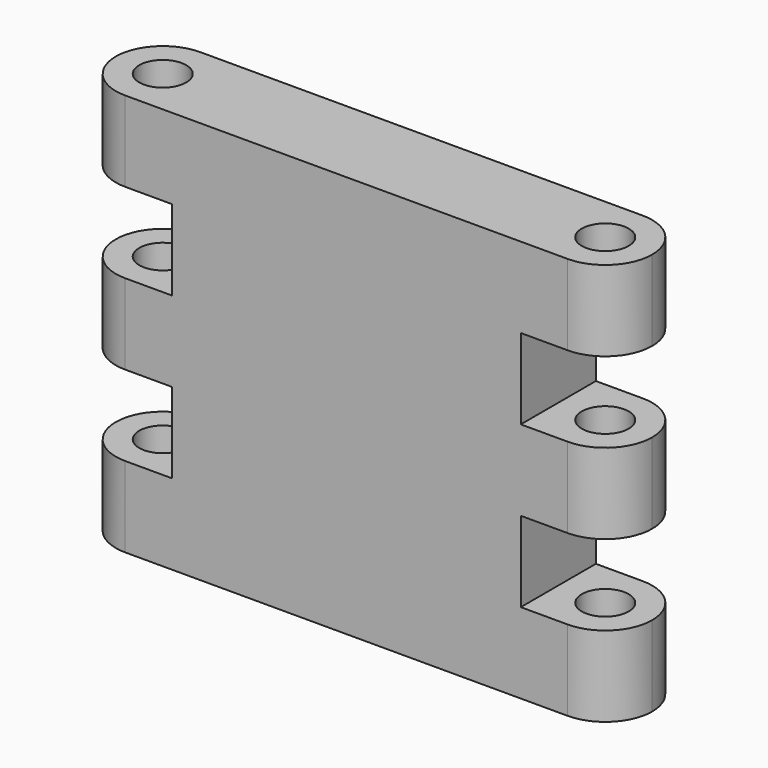
from build123d import *

# Parameters (mm, degrees)
F0_W     = 7
F0_H     = 6
F1_DEPTH = 7
F2_R     = 1.75
F3_DEPTH = 30.001


# Not quite as in the source:
# - a feature names something its author has since deleted; it is built from what else it names


with BuildPart() as f1:
    # F0 (on Front) → F1 (new body)
    with BuildSketch(Plane.XZ):
        with Locations((16.5, 12)):
            Rectangle(F0_W, F0_H)
        with Locations((16.5, -12)):
            Rectangle(F0_W, F0_H)
        with Locations((16.5, 0)):
            Rectangle(F0_W, F0_H)
        with Locations((-16.5, 12)):
            Rectangle(F0_W, F0_H)
        with Locations((-16.5, 0)):
            Rectangle(F0_W, F0_H)
        with Locations((-16.5, -12)):
            Rectangle(F0_W, F0_H)
        Polygon((13, 9), (13, 15), (-13, 15), (-13, 9), (-13, 3), (-13, -3), (-13, -9), (-13, -15), (13, -15), (13, -9), (13, -3), (13, 3), align=None)
    extrude(amount=F1_DEPTH)

    # F2 (on face) → F3 (cut, through all)
    with BuildSketch(Plane(origin=(0, 0, -15), x_dir=(1, 0, 0), z_dir=(0, 0, -1))):
        with Locations((-16.5, 3.5)):
            Circle(F2_R)
        with BuildLine():
            Line((-20, 0), (-16.5, 0))
            ThreePointArc((-16.5, 0), (-18.9748737342, 1.0251262658), (-20, 3.5))
            Line((-20, 3.5), (-20, 0))
        make_face()
        with BuildLine():
            ThreePointArc((-20, 3.5), (-18.9748737342, 5.9748737342), (-16.5, 7))
            Line((-16.5, 7), (-20, 7))
            Line((-20, 7), (-20, 3.5))
        make_face()
        with BuildLine():
            Line((20, 7), (16.5, 7))
            ThreePointArc((16.5, 7), (18.9748737342, 5.9748737342), (20, 3.5))
            Line((20, 3.5), (20, 7))
        make_face()
        with BuildLine():
            ThreePointArc((20, 3.5), (18.9748737342, 1.0251262658), (16.5, 0))
            Line((16.5, 0), (20, 0))
            Line((20, 0), (20, 3.5))
        make_face()
        with Locations((16.5, 3.5)):
            Circle(F2_R)
    extrude(amount=-F3_DEPTH, mode=Mode.SUBTRACT)


solid = f1.part
